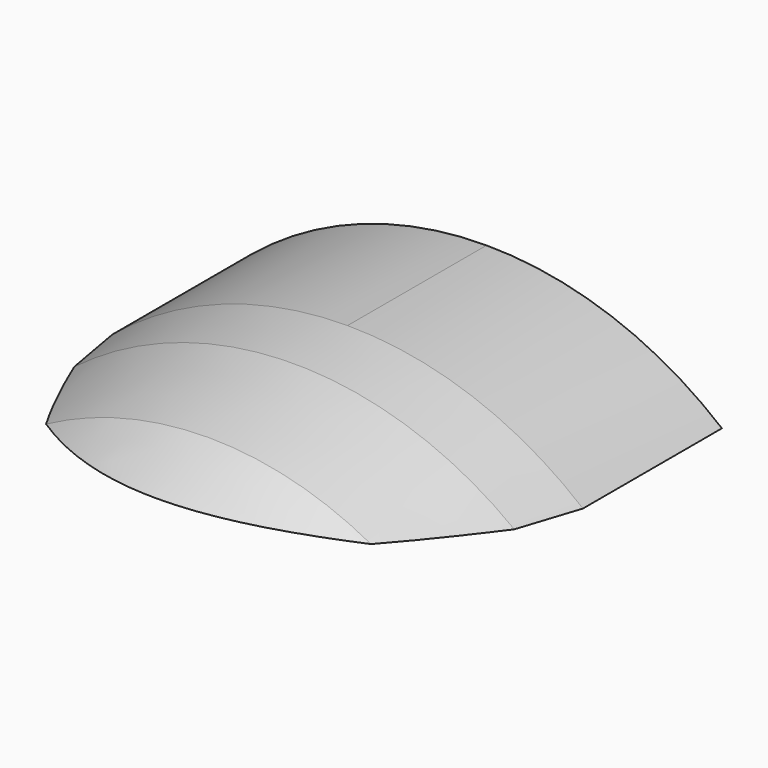
from build123d import *

# Parameters (mm, degrees)
F1_DEPTH    = 75
F2_T2_ANGLE = 123.6693885688
F3_T2_ANGLE = 146.542163671
F4_T2_ANGLE = 137.6625417494
F5_T2_ANGLE = 106.0986339536


# Not quite as in the source:
# - a fillet or chamfer that OpenCascade refuses, or shapes differently, is made with other operations: its cross-section is extruded or revolved along the edge and cut away or added


with BuildPart() as f1:
    # F0 (on Front) → F1 (new body)
    with BuildSketch(Plane.XZ):
        with BuildLine():
            Line((0, 18.0245880038), (0, 8.2237206428))
            ThreePointArc((0, 8.2237206428), (21.1654297157, 6.8979891087), (42, 2.9415184316))
            ThreePointArc((42, 2.9415184316), (22.3131070658, 14.1395036835), (0, 18.0245880038))
        make_face()
        with BuildLine():
            ThreePointArc((-42, 2.9415184316), (-21.1654297157, 6.8979891087), (0, 8.2237206428))
            Line((0, 8.2237206428), (0, 18.0245880038))
            ThreePointArc((0, 18.0245880038), (-22.3131070658, 14.1395036835), (-42, 2.9415184316))
        make_face()
    extrude(amount=F1_DEPTH)

    # F2: chamfer of 10 on 1 edges, made by hand

    # F2_s1 → F2_t2 (revolve, cut)
    with BuildSketch(Plane(origin=(19.9711424115, 0, -37.3002397662), x_dir=(0, 1, 0), z_dir=(0.472017023, 0, -0.8815894339))):
        Polygon((-65, 43.3641317608), (-75, 33.3641317608), (-75, 43.3641317608), align=None)
    revolve(axis=Axis((0, -75, -47.9931074722), (0, -1, 0)), revolution_arc=F2_T2_ANGLE, mode=Mode.SUBTRACT)

    # F3: chamfer of 15 on 1 edges, made by hand

    # F3_s1 → F3_t2 (revolve, cut)
    with BuildSketch(Plane(origin=(13.2298564014, 0, -44.0166808787), x_dir=(0, 1, 0), z_dir=(0.2878439127, 0, -0.9576773371))):
        Polygon((-50, 52.2031716385), (-75.6066017178, 41.5965699207), (-65, 52.2031716385), align=None)
    revolve(axis=Axis((0, -65, -47.9931074722), (0, -1, 0)), revolution_arc=F3_T2_ANGLE, mode=Mode.SUBTRACT)

    # F4: chamfer of 13 on 1 edges, made by hand

    # F4_s1 → F4_t2 (revolve, cut)
    with BuildSketch(Plane(origin=(16.1615809903, 0, -41.7345888895), x_dir=(0, 1, 0), z_dir=(0.3611156728, 0, -0.9325210297))):
        Polygon((-37, 48.6866321803), (-62.0104339226, 43.7117475596), (-50, 48.6866321803), align=None)
    revolve(axis=Axis((0, -50, -47.9931074722), (0, -1, 0)), revolution_arc=F4_T2_ANGLE, mode=Mode.SUBTRACT)

    # F5: chamfer of 6 on 1 edges, made by hand

    # F5_s1 → F5_t2 (revolve, cut)
    with BuildSketch(Plane(origin=(23.0555472536, 0, -30.6506000272), x_dir=(0, 1, 0), z_dir=(0.6011273799, 0, -0.7991532226))):
        Polygon((-31, 37.1677245289), (-42.8847116824, 35.9971825968), (-37, 37.1677245289), align=None)
    revolve(axis=Axis((0, -37, -47.9931074722), (0, -1, 0)), revolution_arc=F5_T2_ANGLE, mode=Mode.SUBTRACT)


solid = f1.part
